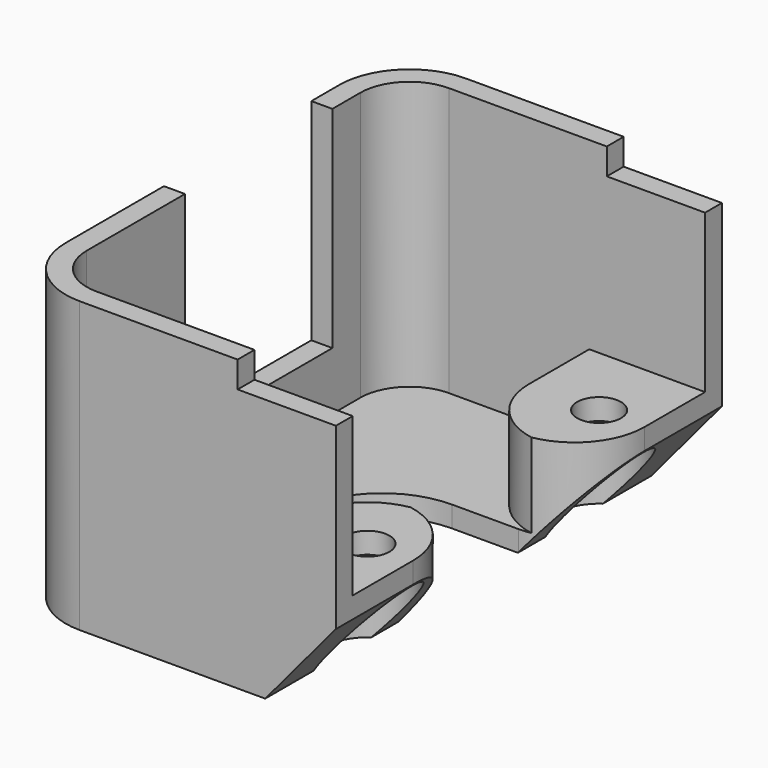
from build123d import *

# Parameters (mm, degrees)
F4_DEPTH       = 13.5
F4_DEPTH_BACK  = 3
F5_R           = 4
F6_T           = -1.2
F7_W           = 6.6
F7_H           = 6
F8_DEPTH       = 13.75
F8_DEPTH_BACK  = 13.75
F3_W           = 8
F3_H           = 8.5
F9_DEPTH       = 4.5
F9_DEPTH_BACK  = 4.3
F11_START      = -6.5
F10_W          = 10.5
F10_H          = 18.4398862173
F11_DEPTH      = 11.4
F12_F1_R       = 4
F12_F2_R       = 4
F12_F3_R       = 4
F12_F4_R       = 4
F0_R           = 1.25
F13_DEPTH      = 7.9
F13_DEPTH_BACK = 7.1
F1_R           = 2.5
F14_DEPTH      = 1.8
F14_DEPTH_BACK = 4.3
F15_R          = 5
F17_DEPTH      = 16
F17_DEPTH_BACK = 16.1
F18_W          = 5.6
F18_H          = 3
F19_DEPTH      = 25
F19_DEPTH_BACK = 25


# Not quite as in the source:
# - a feature names something its author has since deleted; it is built from what else it names


with BuildPart() as f4:
    # F2 (on Top) → F4 (new body, two sides)
    with BuildSketch(Plane.XY) as f4_sk:
        with BuildLine():
            Line((2.6, 4.25), (2.6, 13.75))
            Line((2.6, 13.75), (-16, 13.75))
            Line((-16, 13.75), (-16, -13.75))
            Line((-16, -13.75), (2.6, -13.75))
            Line((2.6, -13.75), (2.6, -4.25))
            Line((2.6, -4.25), (-4.5505102572, -4.25))
            ThreePointArc((-4.5505102572, -4.25), (-8.769806787, -4.7695668459), (-10.3781091101, -0.8343697034))
            Line((-10.3781091101, -0.8343697034), (-9, 4.25))
            Line((-9, 4.25), (2.6, 4.25))
        make_face()
    extrude(amount=F4_DEPTH)
    extrude(f4_sk.sketch, amount=-F4_DEPTH_BACK)

    # F5
    f5_edges = [f4.edges().sort_by_distance(p)[0] for p in [
        (-16, 13.75, 5.25),
        (-16, -13.75, 5.25),
    ]]
    fillet(f5_edges, radius=F5_R)

    # F6
    f6_openings = [f4.faces().sort_by_distance(p)[0] for p in [
        (-4.7, 13.418005, 13.5),
        (2.6, 9, 5.25),
        (2.6, -9, 5.25),
        (-0.975255, -4.25, 5.25),
        (-3.2, 4.25, 5.25),
        (-8.769807, -4.769567, 5.25),
        (-9.689055, 1.707815, 5.25),
    ]]
    offset(amount=F6_T, openings=f6_openings)

    # F7 (on Front) → F8 (join, two sides)
    with BuildSketch(Plane.XZ) as f8_sk:
        with Locations((-0.7, 0)):
            Rectangle(F7_W, F7_H)
    extrude(amount=-F8_DEPTH)
    extrude(f8_sk.sketch, amount=F8_DEPTH_BACK)

    # F3 (on Top) → F9 (cut, two sides)
    with BuildSketch(Plane.XY) as f9_sk:
        with Locations((-1.4, 0)):
            Rectangle(F3_W, F3_H)
    extrude(amount=F9_DEPTH, mode=Mode.SUBTRACT)
    extrude(f9_sk.sketch, amount=-F9_DEPTH_BACK, mode=Mode.SUBTRACT)

    # F10 (on Right) → F11 (cut)
    with BuildSketch(Plane.YZ.offset(F11_START)):
        with Locations((2.5, 10.7199431086)):
            Rectangle(F10_W, F10_H)
    extrude(amount=-F11_DEPTH, mode=Mode.SUBTRACT)

    # F12: fillet of radius 4 on 4 edges, made by hand

    # F12_f1
    f12_f1_edges = [f4.edges().sort_by_distance(p)[0] for p in [
        (-4, -4.25, 0.6),
    ]]
    fillet(f12_f1_edges, radius=F12_F1_R)

    # F12_f2
    f12_f2_edges = [f4.edges().sort_by_distance(p)[0] for p in [
        (-4, 4.25, 0.6),
    ]]
    fillet(f12_f2_edges, radius=F12_F2_R)

    # F12_f3
    f12_f3_edges = [f4.edges().sort_by_distance(p)[0] for p in [
        (2.6, 4.25, 0),
    ]]
    fillet(f12_f3_edges, radius=F12_F3_R)

    # F12_f4
    f12_f4_edges = [f4.edges().sort_by_distance(p)[0] for p in [
        (2.6, -4.25, 0),
    ]]
    fillet(f12_f4_edges, radius=F12_F4_R)

    # F0 (on Top) → F13 (cut, two sides)
    with BuildSketch(Plane.XY) as f13_sk:
        with Locations((0, -8.25)):
            Circle(F0_R)
        with Locations((0, 8.25)):
            Circle(F0_R)
    extrude(amount=F13_DEPTH, mode=Mode.SUBTRACT)
    extrude(f13_sk.sketch, amount=-F13_DEPTH_BACK, mode=Mode.SUBTRACT)

    # F1 (on Top) → F14 (cut, two sides)
    with BuildSketch(Plane.XY) as f14_sk:
        with Locations((0, -8.25)):
            Circle(F1_R)
        with Locations((0, 8.25)):
            Circle(F1_R)
    extrude(amount=F14_DEPTH, mode=Mode.SUBTRACT)
    extrude(f14_sk.sketch, amount=-F14_DEPTH_BACK, mode=Mode.SUBTRACT)

    # F15
    f15_edges = [f4.edges().sort_by_distance(p)[0] for p in [
        (-4.55051, -4.25, -2.4),
        (-9, 4.25, -2.4),
    ]]
    fillet(f15_edges, radius=F15_R)

    # F16 (on Front) → F17 (cut, two sides)
    with BuildSketch(Plane.XZ) as f17_sk:
        Polygon((2.6, 1.8), (-4.0077234488, -6.074778159), (2.3954068281, -10.9375437775), (8.7053719483, -6.2603745918), align=None)
    extrude(amount=F17_DEPTH, mode=Mode.SUBTRACT)
    extrude(f17_sk.sketch, amount=-F17_DEPTH_BACK, mode=Mode.SUBTRACT)

    # F18 (on Front) → F19 (cut, two sides)
    with BuildSketch(Plane.XZ) as f19_sk:
        with Locations((-0.2, 13.5)):
            Rectangle(F18_W, F18_H)
    extrude(amount=F19_DEPTH, mode=Mode.SUBTRACT)
    extrude(f19_sk.sketch, amount=-F19_DEPTH_BACK, mode=Mode.SUBTRACT)


solid = f4.part
